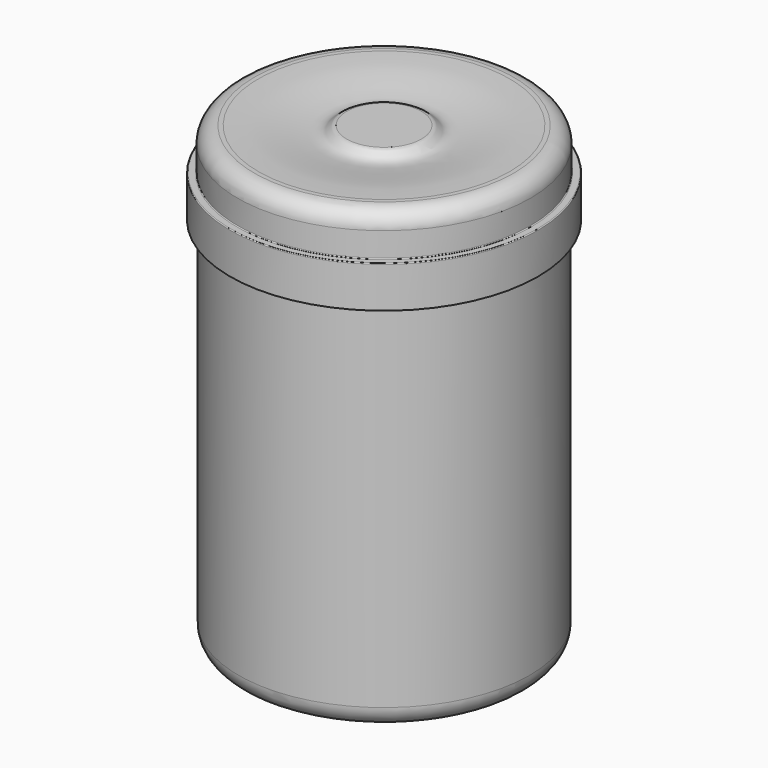
from build123d import *

# Parameters (mm, degrees)
F2_W = 15
F2_H = 4


# Not quite as in the source:
# - ends of sketch curves that miss each other by under 0.0002 mm in the source are joined


with BuildPart() as f1:
    # F0 (on Front) → F1 (revolve)
    with BuildSketch(Plane.XZ):
        with BuildLine():
            Line((350, -950), (350, 0))
            Line((350, 0), (0, 0))
            Line((0, 0), (0, -1000))
            Line((0, -1000), (300, -1000))
            ThreePointArc((300, -1000), (335.3553390593, -985.3553390593), (350, -950))
        make_face()
    revolve(axis=Axis((0, 0, -563.781440258), (0, 0, 1)))

    # F2 (on Front) → F3 (revolve)
    with BuildSketch(Plane.XZ):
        with Locations((357.5, -2)):
            Rectangle(F2_W, F2_H)
    revolve(axis=Axis((0, 0, -500), (0, 0, 1)))


with BuildPart() as f5:
    # F4 (on Front) → F5 (revolve)
    with BuildSketch(Plane.XZ):
        with BuildLine():
            Line((368, 0), (354, 0))
            ThreePointArc((354, 0), (352.5857864376, 0.5857864376), (352, 2))
            Line((352, 2), (352, 60))
            ThreePointArc((352, 60), (340.2842712475, 88.2842712475), (312, 100))
            Line((312, 100), (302, 100))
            add(Edge.make_bspline(
                [(90, 100), (99.4711880321, 100), (108.4193994424, 84.3913848943), (139.1428176435, 80.5684134054), (181.851883894, 89.2072392235), (234.6883361244, 96.2560851887), (267.4291003084, 100), (302, 100)],
                knots=[2.85798e-05, 2.85798e-05, 2.85798e-05, 2.85798e-05, 0.1499893339, 0.3139008613, 0.5198138943, 0.7376397347, 1, 1, 1, 1], degree=3))
            add(Edge.make_bspline(
                [(89.994584319, 99.9999991873), (89.9963897347, 99.9999997291), (89.9981949617, 100), (90, 100)],
                knots=[0, 0, 0, 0, 2.85798e-05, 2.85798e-05, 2.85798e-05, 2.85798e-05], degree=3))
            Line((89.994584319, 99.9999991873), (0, 100))
            Line((0, 100), (0, -100))
            Line((0, -100), (370, -100))
            Line((370, -100), (370, -2))
            ThreePointArc((370, -2), (369.4142135624, -0.5857864376), (368, 0))
        make_face()
    revolve(axis=Axis((0, 0, 0), (0, 0, 1)))


solid = Compound([f1.part, f5.part])
